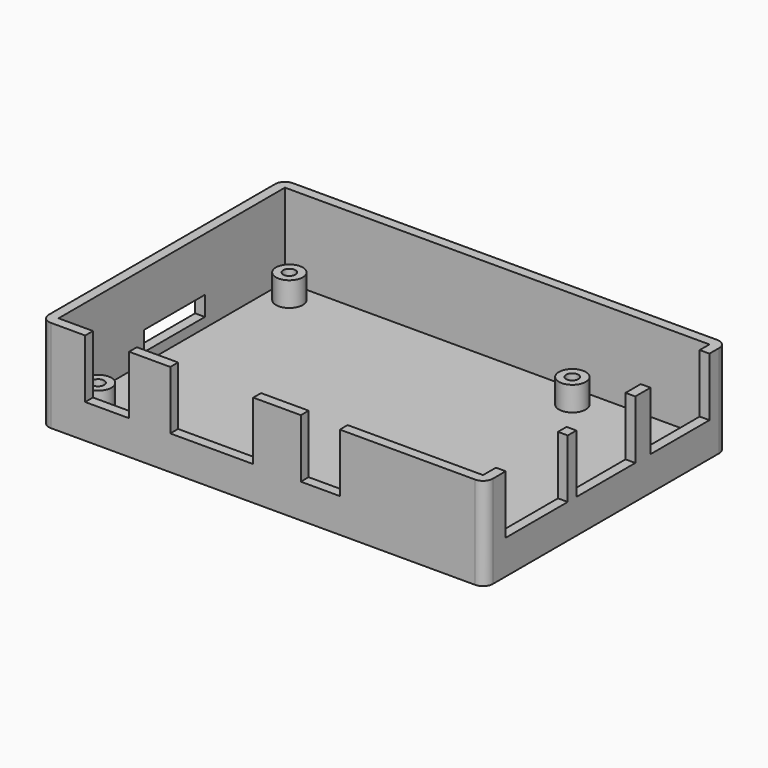
from build123d import *

# Parameters (mm, degrees)
F0_W           = 91
F0_H           = 62
F0_W_2         = 87
F0_H_2         = 58
F1_DEPTH       = 2
F2_DEPTH       = 19
F3_R           = 2.75
F3_R_2         = 1.25
F4_DEPTH       = 5
F5_DEPTH       = 2.001
F6_W           = 3
F6_H           = 15.1
F6_H_2         = 15.9
F6_W_2         = 9
F6_H_3         = 2
F6_W_3         = 17
F6_W_4         = 8
F7_DEPTH       = 12
F8_R           = 2
F9_W           = 2
F9_H           = 15.6
F10_DEPTH      = 3
F10_DEPTH_BACK = 1


# Not quite as in the source:
# - a feature names something its author has since deleted; it is built from what else it names


with BuildPart() as f1:
    # F0 (on Top) → F1 (new body)
    with BuildSketch(Plane.XY):
        with Locations((45.5, 31)):
            Rectangle(F0_W, F0_H)
        with Locations((45.5, 31)):
            Rectangle(F0_W_2, F0_H_2, mode=Mode.SUBTRACT)
        with Locations((45.5, 31)):
            Rectangle(F0_W_2, F0_H_2)
    extrude(amount=F1_DEPTH)

    # F0 (on Top) → F2 (join)
    with BuildSketch(Plane.XY):
        with Locations((45.5, 31)):
            Rectangle(F0_W, F0_H)
        with Locations((45.5, 31)):
            Rectangle(F0_W_2, F0_H_2, mode=Mode.SUBTRACT)
    extrude(amount=F2_DEPTH)

    # F3 (on face) → F4 (join)
    with BuildSketch(Plane.XY.offset(2)):
        with Locations((6.5, 55.5)):
            Circle(F3_R)
        with Locations((6.5, 55.5)):
            Circle(F3_R_2, mode=Mode.SUBTRACT)
        with Locations((64.5, 55.5)):
            Circle(F3_R)
        with Locations((64.5, 55.5)):
            Circle(F3_R_2, mode=Mode.SUBTRACT)
        with Locations((64.5, 6.5)):
            Circle(F3_R)
        with Locations((64.5, 6.5)):
            Circle(F3_R_2, mode=Mode.SUBTRACT)
        with Locations((6.5, 6.5)):
            Circle(F3_R)
        with Locations((6.5, 6.5)):
            Circle(F3_R_2, mode=Mode.SUBTRACT)
    extrude(amount=F4_DEPTH)

    # F5 (cut, through all): faces of the model
    f5_faces = [f1.faces().sort_by_distance(p)[0] for p in [
        (6.5, 55.5, 2),
        (64.5, 55.5, 2),
        (64.5, 6.5, 2),
        (6.5, 6.5, 2),
    ]]
    extrude(f5_faces, amount=-F5_DEPTH, mode=Mode.SUBTRACT)

    # F6 (on face) → F7 (cut, through all)
    with BuildSketch(Plane.XY.offset(19)):
        with Locations((89.5, 49.95)):
            Rectangle(F6_W, F6_H)
        with Locations((89.5, 30.95)):
            Rectangle(F6_W, F6_H)
        with Locations((89.5, 13.25)):
            Rectangle(F6_W, F6_H_2)
        with Locations((13.55, 1)):
            Rectangle(F6_W_2, F6_H_3)
        with Locations((35, 1)):
            Rectangle(F6_W_3, F6_H_3)
        with Locations((57.25, 1)):
            Rectangle(F6_W_4, F6_H_3)
    extrude(amount=-F7_DEPTH, mode=Mode.SUBTRACT)

    # F8
    f8_edges = [f1.edges().sort_by_distance(p)[0] for p in [
        (91, 0, 9.5),
        (91, 62, 9.5),
        (0, 0, 9.5),
        (0, 62, 9.5),
    ]]
    fillet(f8_edges, radius=F8_R)

    # F9 (on face) → F10 (cut, two sides)
    with BuildSketch(Plane.XY.offset(7)) as f10_sk:
        with Locations((1, 31.7)):
            Rectangle(F9_W, F9_H)
    extrude(amount=-F10_DEPTH, mode=Mode.SUBTRACT)
    extrude(f10_sk.sketch, amount=F10_DEPTH_BACK, mode=Mode.SUBTRACT)


solid = f1.part
